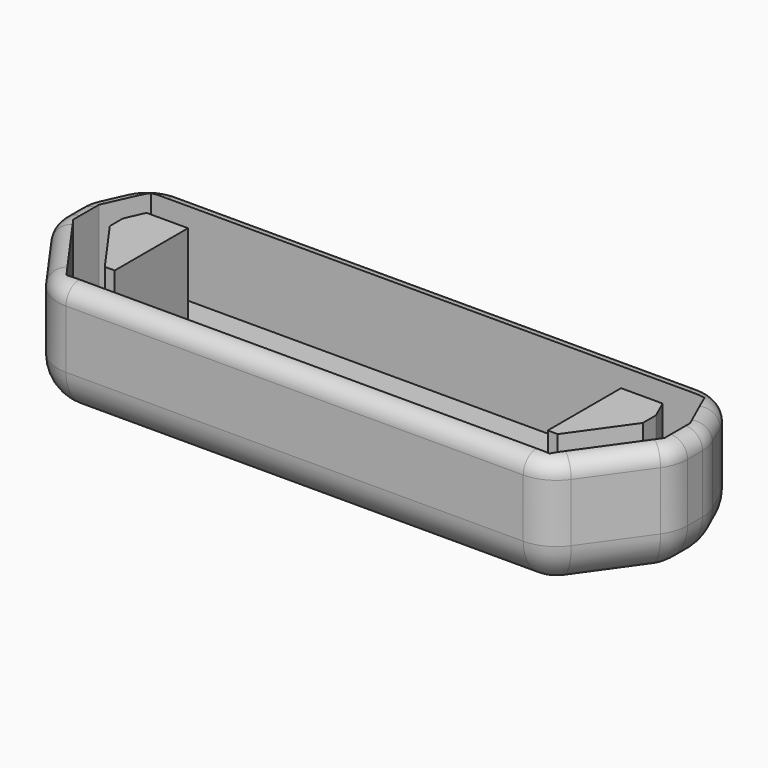
from build123d import *

# Parameters (mm, degrees)
F1_DEPTH     = 5
F3_DEPTH     = 2
F4_R         = 2.5
F5_T1_DEPTH  = 27.4519311484
F5_T3_DEPTH  = 1.45667481
F5_T5_DEPTH  = 1.1206167057
F5_T7_DEPTH  = 31.3076734299
F5_T9_DEPTH  = 4.3560651868
F5_T11_DEPTH = 1.45667481
F5_T13_DEPTH = 4.3560651868
F5_T16_ANGLE = 24.1585538769
F5_T18_ANGLE = 65.8414461231
F5_T20_ANGLE = 35.4104549915
F5_T22_ANGLE = 65.8414461231
F5_T24_ANGLE = 54.5895450085
F5_T26_ANGLE = 24.1585538769
F5_T28_ANGLE = 54.5895450085
F5_T30_ANGLE = 35.4104549915


# Not quite as in the source:
# - a fillet or chamfer that OpenCascade refuses, or shapes differently, is made with other operations: its cross-section is extruded or revolved along the edge and cut away or added


with BuildPart() as f1:
    # F0 (on Top) → F1 (new body)
    with BuildSketch(Plane.XY):
        Polygon((18.75, 6.7059138706), (17.27244219, 10), (0, 10), (-17.27244219, 10), (-18.75, 6.7059138706), (-18.75, 4.2521861975), (-15.0160229505, -1), (0, -1), (15.0160229505, -1), (18.75, 4.2521861975), align=None)
        Polygon((14.5, 0), (0, 0), (-14.5, 0), (-17.75, 4.5714274394), (-17.75, 6.4919107255), (-16.625, 9), (0, 9), (16.625, 9), (17.75, 6.4919107255), (17.75, 4.5714274394), align=None, mode=Mode.SUBTRACT)
    extrude(amount=F1_DEPTH)



with BuildPart() as f1b:
    # F0 (on Top) → F1, piece 2 (new body)
    with BuildSketch(Plane.XY):
        Polygon((-15.4919761674, 7.25), (-16, 6.1174052217), (-16, 5.1300996126), (-13.5969598365, 1.75), (-13, 1.75), (-13, 7.25), align=None)
    extrude(amount=F1_DEPTH)


with BuildPart() as f1c:
    # F0 (on Top) → F1, piece 3 (new body)
    with BuildSketch(Plane.XY):
        Polygon((16, 6.1174052217), (15.4919761674, 7.25), (13, 7.25), (13, 1.75), (13.5969598365, 1.75), (16, 5.1300996126), align=None)
    extrude(amount=F1_DEPTH)


with BuildPart() as f1_1:
    add(f1.part)

    add(f1b.part)  # F3 merges F1b

    add(f1c.part)  # F3 merges F1c
    # F2 (on face) → F3 (join)
    with BuildSketch(Plane(origin=(0, 0, 0), x_dir=(1, 0, 0), z_dir=(0, 0, -1))):
        Polygon((-17.27244219, -10), (17.27244219, -10), (18.75, -6.7059138706), (18.75, -4.2521861975), (15.0160229505, 1), (-15.0160229505, 1), (-18.75, -4.2521861975), (-18.75, -6.7059138706), align=None)
    extrude(amount=F3_DEPTH)

    # F4
    f4_edges = [f1_1.edges().sort_by_distance(p)[0] for p in [
        (-18.75, 5.47905, -2),
        (-18.011221, 8.352957, -2),
        (0, 10, -2),
        (18.011221, 8.352957, -2),
        (18.75, 5.47905, -2),
        (16.883011, 1.626093, -2),
        (0, -1, -2),
        (-16.883011, 1.626093, -2),
        (-15.016023, -1, 1.5),
        (-18.75, 4.252186, 1.5),
        (-18.75, 6.705914, 1.5),
        (-17.272442, 10, 1.5),
        (15.016023, -1, 1.5),
        (18.75, 4.252186, 1.5),
        (17.272442, 10, 1.5),
        (18.75, 6.705914, 1.5),
    ]]
    fillet(f4_edges, radius=F4_R)

    # F5: fillet of radius 1 on 16 edges, made by hand

    # F5_s2 → F5_t1 (cut)
    with BuildSketch(Plane.YZ.offset(-13.7259655742)):
        with BuildLine():
            ThreePointArc((0, 5), (-0.7071067812, 4.7071067812), (-1, 4))
            Line((-1, 4), (-1, 5))
            Line((-1, 5), (0, 5))
        make_face()
    extrude(amount=F5_T1_DEPTH, mode=Mode.SUBTRACT)

    # F5_s4 → F5_t3 (cut)
    with BuildSketch(Plane(origin=(0.417485186, -0.9307467709, 0), x_dir=(0, 0, 1), z_dir=(-0.4092631251, 0.9124164041, 0))):
        with BuildLine():
            ThreePointArc((4, 19.8522908438), (4.7071067812, 19.5593976249), (5, 18.8522908438))
            Line((5, 18.8522908438), (5, 19.8522908438))
            Line((5, 19.8522908438), (4, 19.8522908438))
        make_face()
    extrude(amount=F5_T3_DEPTH, mode=Mode.SUBTRACT)

    # F5_s6 → F5_t5 (cut)
    with BuildSketch(Plane.XZ.offset(-6.1709060079)):
        with BuildLine():
            ThreePointArc((17.75, 5), (18.4571067812, 4.7071067812), (18.75, 4))
            Line((18.75, 4), (18.75, 5))
            Line((18.75, 5), (17.75, 5))
        make_face()
        with BuildLine():
            ThreePointArc((-17.75, 5), (-18.4571067812, 4.7071067812), (-18.75, 4))
            Line((-18.75, 4), (-18.75, 5))
            Line((-18.75, 5), (-17.75, 5))
        make_face()
    extrude(amount=F5_T5_DEPTH, mode=Mode.SUBTRACT)

    # F5_s8 → F5_t7 (cut)
    with BuildSketch(Plane.YZ.offset(-15.6538367149)):
        with BuildLine():
            ThreePointArc((9, 5), (9.7071067812, 4.7071067812), (10, 4))
            Line((10, 4), (10, 5))
            Line((10, 5), (9, 5))
        make_face()
    extrude(amount=F5_T7_DEPTH, mode=Mode.SUBTRACT)

    # F5_s10 → F5_t9 (cut)
    with BuildSketch(Plane(origin=(5.3167143619, 7.4784535142, 0), x_dir=(0, 0, 1), z_dir=(0.5794299023, 0.8150220784, 0))):
        with BuildLine():
            ThreePointArc((5, 11.8178201367), (4.7071067812, 12.5249269179), (4, 12.8178201367))
            Line((4, 12.8178201367), (5, 12.8178201367))
            Line((5, 12.8178201367), (5, 11.8178201367))
        make_face()
    extrude(amount=F5_T9_DEPTH, mode=Mode.SUBTRACT)

    # F5_s12 → F5_t11 (cut)
    with BuildSketch(Plane(origin=(0.1786780991, 0.3983472212, 0), x_dir=(0, 0, 1), z_dir=(-0.4092631251, -0.9124164041, 0))):
        with BuildLine():
            ThreePointArc((5, 18.8522908438), (4.7071067812, 19.5593976249), (4, 19.8522908438))
            Line((4, 19.8522908438), (5, 19.8522908438))
            Line((5, 19.8522908438), (5, 18.8522908438))
        make_face()
    extrude(amount=F5_T11_DEPTH, mode=Mode.SUBTRACT)

    # F5_s14 → F5_t13 (cut)
    with BuildSketch(Plane(origin=(-7.8407487877, 11.0287428164, 0), x_dir=(0, 0, 1), z_dir=(0.5794299023, -0.8150220784, 0))):
        with BuildLine():
            ThreePointArc((5, 11.8178201367), (4.7071067812, 12.5249269179), (4, 12.8178201367))
            Line((4, 12.8178201367), (5, 12.8178201367))
            Line((5, 12.8178201367), (5, 11.8178201367))
        make_face()
    extrude(amount=F5_T13_DEPTH, mode=Mode.SUBTRACT)

    # F5_s15 → F5_t16 (revolve, cut)
    with BuildSketch(Plane(origin=(0.417485186, -0.9307467709, 0), x_dir=(0, 0, 1), z_dir=(-0.4092631251, 0.9124164041, 0))):
        with BuildLine():
            ThreePointArc((5, 18.8522908438), (4.7071067812, 19.5593976249), (4, 19.8522908438))
            Line((4, 19.8522908438), (5, 19.8522908438))
            Line((5, 19.8522908438), (5, 18.8522908438))
        make_face()
    revolve(axis=Axis((16.25, 6.1709060079, 5), (0, 0, -1)), revolution_arc=F5_T16_ANGLE, mode=Mode.SUBTRACT)

    # F5_s17 → F5_t18 (revolve, cut)
    with BuildSketch(Plane(origin=(-0.1786780991, 0.3983472212, 0), x_dir=(0, 0, 1), z_dir=(0.4092631251, -0.9124164041, 0))):
        with BuildLine():
            ThreePointArc((5, -18.8522908438), (4.7071067812, -19.5593976249), (4, -19.8522908438))
            Line((4, -19.8522908438), (5, -19.8522908438))
            Line((5, -19.8522908438), (5, -18.8522908438))
        make_face()
    revolve(axis=Axis((15.6538367149, 7.5, 5), (0, 0, 1)), revolution_arc=F5_T18_ANGLE, mode=Mode.SUBTRACT)

    # F5_s19 → F5_t20 (revolve, cut)
    with BuildSketch(Plane.XZ.offset(-5.0502893022)):
        with BuildLine():
            ThreePointArc((17.75, 5), (18.4571067812, 4.7071067812), (18.75, 4))
            Line((18.75, 4), (18.75, 5))
            Line((18.75, 5), (17.75, 5))
        make_face()
    revolve(axis=Axis((16.25, 5.0502893022, 5), (0, 0, -1)), revolution_arc=F5_T20_ANGLE, mode=Mode.SUBTRACT)

    # F5_s21 → F5_t22 (revolve, cut)
    with BuildSketch(Plane.YZ.offset(-15.6538367149)):
        with BuildLine():
            ThreePointArc((9, 5), (9.7071067812, 4.7071067812), (10, 4))
            Line((10, 4), (10, 5))
            Line((10, 5), (9, 5))
        make_face()
    revolve(axis=Axis((-15.6538367149, 7.5, 5), (0, 0, 1)), revolution_arc=F5_T22_ANGLE, mode=Mode.SUBTRACT)

    # F5_s23 → F5_t24 (revolve, cut)
    with BuildSketch(Plane(origin=(5.3167143619, 7.4784535142, 0), x_dir=(0, 0, 1), z_dir=(0.5794299023, 0.8150220784, 0))):
        with BuildLine():
            ThreePointArc((5, 11.8178201367), (4.7071067812, 12.5249269179), (4, 12.8178201367))
            Line((4, 12.8178201367), (5, 12.8178201367))
            Line((5, 12.8178201367), (5, 11.8178201367))
        make_face()
    revolve(axis=Axis((13.7259655742, 1.5, 5), (0, 0, -1)), revolution_arc=F5_T24_ANGLE, mode=Mode.SUBTRACT)

    # F5_s25 → F5_t26 (revolve, cut)
    with BuildSketch(Plane(origin=(-0.417485186, -0.9307467709, 0), x_dir=(0, 0, 1), z_dir=(0.4092631251, 0.9124164041, 0))):
        with BuildLine():
            ThreePointArc((5, -18.8522908438), (4.7071067812, -19.5593976249), (4, -19.8522908438))
            Line((4, -19.8522908438), (5, -19.8522908438))
            Line((5, -19.8522908438), (5, -18.8522908438))
        make_face()
    revolve(axis=Axis((-16.25, 6.1709060079, 5), (0, 0, 1)), revolution_arc=F5_T26_ANGLE, mode=Mode.SUBTRACT)

    # F5_s27 → F5_t28 (revolve, cut)
    with BuildSketch(Plane(origin=(-5.3167143619, 7.4784535142, 0), x_dir=(0, 0, 1), z_dir=(-0.5794299023, 0.8150220784, 0))):
        with BuildLine():
            ThreePointArc((5, -11.8178201367), (4.7071067812, -12.5249269179), (4, -12.8178201367))
            Line((4, -12.8178201367), (5, -12.8178201367))
            Line((5, -12.8178201367), (5, -11.8178201367))
        make_face()
    revolve(axis=Axis((-13.7259655742, 1.5, 5), (0, 0, 1)), revolution_arc=F5_T28_ANGLE, mode=Mode.SUBTRACT)

    # F5_s29 → F5_t30 (revolve, cut)
    with BuildSketch(Plane.XZ.offset(-5.0502893022)):
        with BuildLine():
            ThreePointArc((-17.75, 5), (-18.4571067812, 4.7071067812), (-18.75, 4))
            Line((-18.75, 4), (-18.75, 5))
            Line((-18.75, 5), (-17.75, 5))
        make_face()
    revolve(axis=Axis((-16.25, 5.0502893022, 5), (0, 0, 1)), revolution_arc=F5_T30_ANGLE, mode=Mode.SUBTRACT)


solid = f1_1.part
